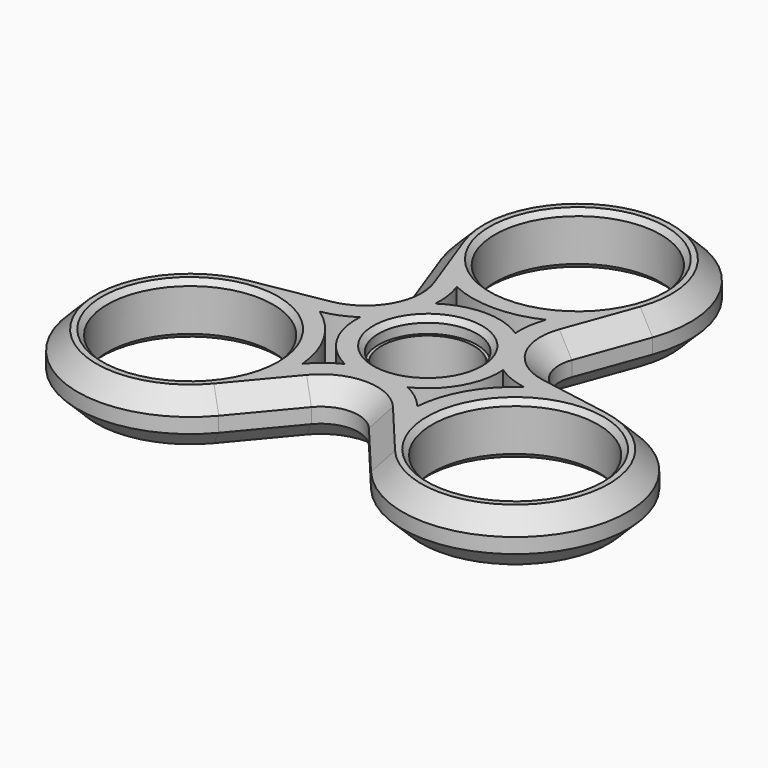
from build123d import *

# Parameters (mm, degrees)
F0_R     = 11.05
F0_R_2   = 6.55
F1_DEPTH = 7
F2_R     = 5
F3_SIZE  = 2.5
F4_R     = 6.55
F4_R_2   = 6.15
F5_DEPTH = 5
F6_SIZE  = 0.7
F8_DEPTH = 25


with BuildPart() as f1:
    # F0 (on Top) → F1 (new body)
    with BuildSketch(Plane.XY):
        with BuildLine():
            Line((8.6602540378, 5), (14.0883655764, 19.8504412435))
            ThreePointArc((14.0883655764, 19.8504412435), (0, 40), (-14.0883655764, 19.8504412435))
            Line((-14.0883655764, 19.8504412435), (-8.6602540378, 5))
            Line((-8.6602540378, 5), (-24.2351691813, 2.2756618652))
            ThreePointArc((-24.2351691813, 2.2756618652), (-34.6410161514, -20), (-10.146803605, -22.1261031087))
            Line((-10.146803605, -22.1261031087), (0, -10))
            Line((0, -10), (10.146803605, -22.1261031087))
            ThreePointArc((10.146803605, -22.1261031087), (34.6410161514, -20), (24.2351691813, 2.2756618652))
            Line((24.2351691813, 2.2756618652), (8.6602540378, 5))
        make_face()
        with Locations((-21.6506350946, -12.5)):
            Circle(F0_R, mode=Mode.SUBTRACT)
        with Locations((21.6506350946, -12.5)):
            Circle(F0_R, mode=Mode.SUBTRACT)
        Circle(F0_R_2, mode=Mode.SUBTRACT)
        with Locations((0, 25)):
            Circle(F0_R, mode=Mode.SUBTRACT)
    extrude(amount=F1_DEPTH)

    # F2
    f2_edges = [f1.edges().sort_by_distance(p)[0] for p in [
        (0, -10, 3.5),
        (8.660254, 5, 3.5),
        (-8.660254, 5, 3.5),
    ]]
    fillet(f2_edges, radius=F2_R)

    # F3
    f3_edges = [f1.edges().sort_by_distance(p)[0] for p in [
        (-19.390694, 3.123049, 7),
        (-6.990707, -18.354358, 0),
        (12.399987, 15.231309, 0),
        (12.399987, 15.231309, 7),
        (11.077604, 6.395657, 0),
        (0, 40, 0),
        (19.390694, 3.123049, 0),
        (-12.399987, 15.231309, 0),
        (34.641016, -20, 0),
        (-11.077604, 6.395657, 0),
        (6.990707, -18.354358, 0),
        (-19.390694, 3.123049, 0),
        (0, -12.791315, 0),
        (-34.641016, -20, 0),
        (11.077604, 6.395657, 7),
        (0, 40, 7),
        (19.390694, 3.123049, 7),
        (-12.399987, 15.231309, 7),
        (34.641016, -20, 7),
        (-11.077604, 6.395657, 7),
        (6.990707, -18.354358, 7),
        (0, -12.791315, 7),
        (-34.641016, -20, 7),
        (-6.990707, -18.354358, 7),
    ]]
    chamfer(f3_edges, length=F3_SIZE)

    # F4 (on face) → F5 (join)
    with BuildSketch(Plane(origin=(0, 0, 0), x_dir=(1, 0, 0), z_dir=(0, 0, -1))):
        Circle(F4_R)
        Circle(F4_R_2, mode=Mode.SUBTRACT)
    extrude(amount=-F5_DEPTH)

    # F6
    f6_edges = [f1.edges().sort_by_distance(p)[0] for p in [
        (-6.55, 0, 7),
        (-32.700635, -12.5, 7),
        (10.600635, -12.5, 7),
        (-11.05, 25, 7),
        (-32.700635, -12.5, 0),
        (10.600635, -12.5, 0),
        (-11.05, 25, 0),
    ]]
    chamfer(f6_edges, length=F6_SIZE)

    # F7 (on face) → F8 (cut)
    with BuildSketch(Plane.XY.offset(7)):
        with BuildLine():
            ThreePointArc((-4.1925255318, -8.5805145338), (-8.2705426061, -4.775), (-9.5272063297, 0.6594236504))
            ThreePointArc((-9.5272063297, 0.6594236504), (-11.4782376336, -0.3808245165), (-13.6062935442, -0.9808390488))
            ThreePointArc((-13.6062935442, -0.9808390488), (-9.4829781714, -5.475), (-7.6525783054, -11.2929763362))
            ThreePointArc((-7.6525783054, -11.2929763362), (-6.0689225225, -9.7500331232), (-4.1925255318, -8.5805145338))
        make_face()
        with BuildLine():
            ThreePointArc((-5.3346807979, 7.9210908835), (0, 9.55), (5.3346807979, 7.9210908835))
            ThreePointArc((5.3346807979, 7.9210908835), (5.4093151112, 10.1308576396), (5.9537152388, 12.273815385))
            ThreePointArc((5.9537152388, 12.273815385), (0, 10.95), (-5.9537152388, 12.273815385))
            ThreePointArc((-5.9537152388, 12.273815385), (-5.4093151112, 10.1308576396), (-5.3346807979, 7.9210908835))
        make_face()
        with BuildLine():
            ThreePointArc((9.5272063297, 0.6594236504), (8.2705426061, -4.775), (4.1925255318, -8.5805145338))
            ThreePointArc((4.1925255318, -8.5805145338), (6.0689225225, -9.7500331232), (7.6525783054, -11.2929763362))
            ThreePointArc((7.6525783054, -11.2929763362), (9.4829781714, -5.475), (13.6062935442, -0.9808390488))
            ThreePointArc((13.6062935442, -0.9808390488), (11.4782376336, -0.3808245165), (9.5272063297, 0.6594236504))
        make_face()
    extrude(amount=-F8_DEPTH, mode=Mode.SUBTRACT)


solid = f1.part
